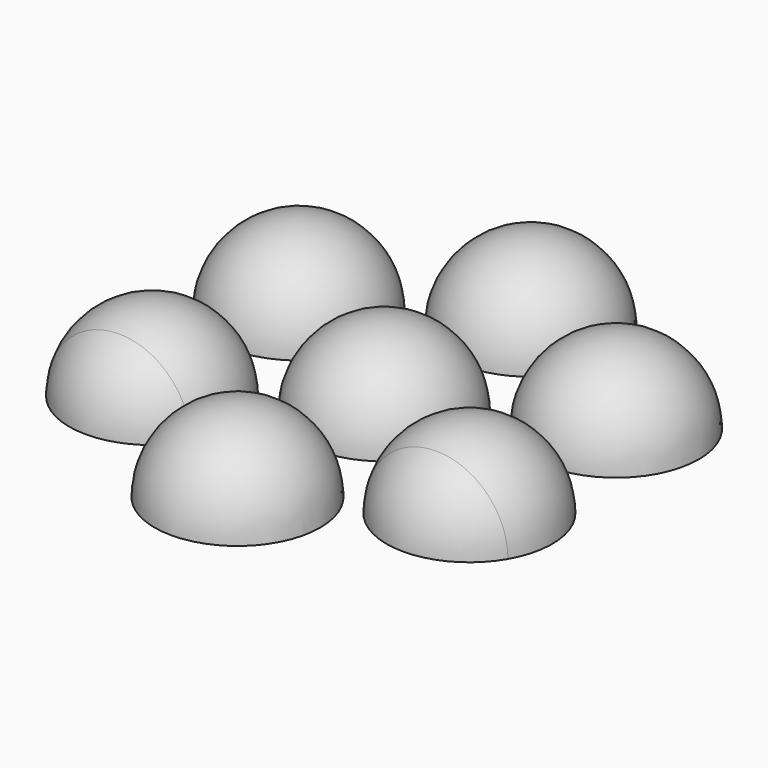
from build123d import *

# Parameters (mm, degrees)
F1_ANGLE = 180
F3_ANGLE = 180
F4_ANGLE = 180
F5_ANGLE = 180


with BuildPart() as f1:
    # F0 (on Top) → F1 (revolve)
    with BuildSketch(Plane.XY):
        with BuildLine():
            Line((0, -4.7), (0, 4.7))
            ThreePointArc((0, 4.7), (-4.7, 0), (0, -4.7))
        make_face()
    revolve(axis=Axis((0, 0, 0), (0, 1, 0)), revolution_arc=F1_ANGLE)


with BuildPart() as f3:
    # F2 (on Top) → F3 (revolve)
    with BuildSketch(Plane.XY):
        with BuildLine():
            ThreePointArc((0, 5.7), (4.7, 10.4), (0, 15.1))
            Line((0, 15.1), (0, 5.7))
        make_face()
    revolve(axis=Axis((0, 10.4, 0), (0, -1, 0)), revolution_arc=F3_ANGLE)


with BuildPart() as f3b:
    # F2 (on Top) → F3, piece 2 (revolve)
    with BuildSketch(Plane.XY):
        with BuildLine():
            ThreePointArc((0, -15.1), (4.7, -10.4), (0, -5.7))
            Line((0, -5.7), (0, -15.1))
        make_face()
    revolve(axis=Axis((0, 10.4, 0), (0, -1, 0)), revolution_arc=F3_ANGLE)


with BuildPart() as f4:
    # F2 (on Top) → F4 (revolve)
    with BuildSketch(Plane.XY):
        with BuildLine():
            Line((-9.0066641994, -5.2), (-9.0066641994, -0.5))
            ThreePointArc((-9.0066641994, -0.5), (-13.0769835971, -2.85), (-13.0769835971, -7.55))
            Line((-13.0769835971, -7.55), (-9.0066641994, -5.2))
        make_face()
        with BuildLine():
            Line((-9.0066641994, -9.9), (-9.0066641994, -5.2))
            Line((-9.0066641994, -5.2), (-13.0769835971, -7.55))
            ThreePointArc((-13.0769835971, -7.55), (-11.3566641994, -9.2703193978), (-9.0066641994, -9.9))
        make_face()
    revolve(axis=Axis((-9.0066641994, 5.2, 0), (0, 1, 0)), revolution_arc=F4_ANGLE)


with BuildPart() as f4b:
    # F2 (on Top) → F4, piece 2 (revolve)
    with BuildSketch(Plane.XY):
        with BuildLine():
            Line((-9.0066641994, 0.5), (-9.0066641994, 9.9))
            ThreePointArc((-9.0066641994, 9.9), (-13.7066641994, 5.2), (-9.0066641994, 0.5))
        make_face()
    revolve(axis=Axis((-9.0066641994, 5.2, 0), (0, 1, 0)), revolution_arc=F4_ANGLE)


with BuildPart() as f5:
    # F2 (on Top) → F5 (revolve)
    with BuildSketch(Plane.XY):
        with BuildLine():
            ThreePointArc((9.0066641994, 0.5), (13.7066641994, 5.2), (9.0066641994, 9.9))
            Line((9.0066641994, 9.9), (9.0066641994, 0.5))
        make_face()
    revolve(axis=Axis((9.0066641994, 5.2, 0), (0, -1, 0)), revolution_arc=F5_ANGLE)


with BuildPart() as f5b:
    # F2 (on Top) → F5, piece 2 (revolve)
    with BuildSketch(Plane.XY):
        with BuildLine():
            Line((13.0769835971, -7.55), (9.0066641994, -5.2))
            Line((9.0066641994, -5.2), (9.0066641994, -9.9))
            ThreePointArc((9.0066641994, -9.9), (11.3566641994, -9.2703193978), (13.0769835971, -7.55))
        make_face()
        with BuildLine():
            ThreePointArc((13.0769835971, -7.55), (13.0769835971, -2.85), (9.0066641994, -0.5))
            Line((9.0066641994, -0.5), (9.0066641994, -5.2))
            Line((9.0066641994, -5.2), (13.0769835971, -7.55))
        make_face()
    revolve(axis=Axis((9.0066641994, 5.2, 0), (0, -1, 0)), revolution_arc=F5_ANGLE)


solid = Compound([f1.part, f3.part, f3b.part, f4.part, f4b.part, f5.part, f5b.part])
